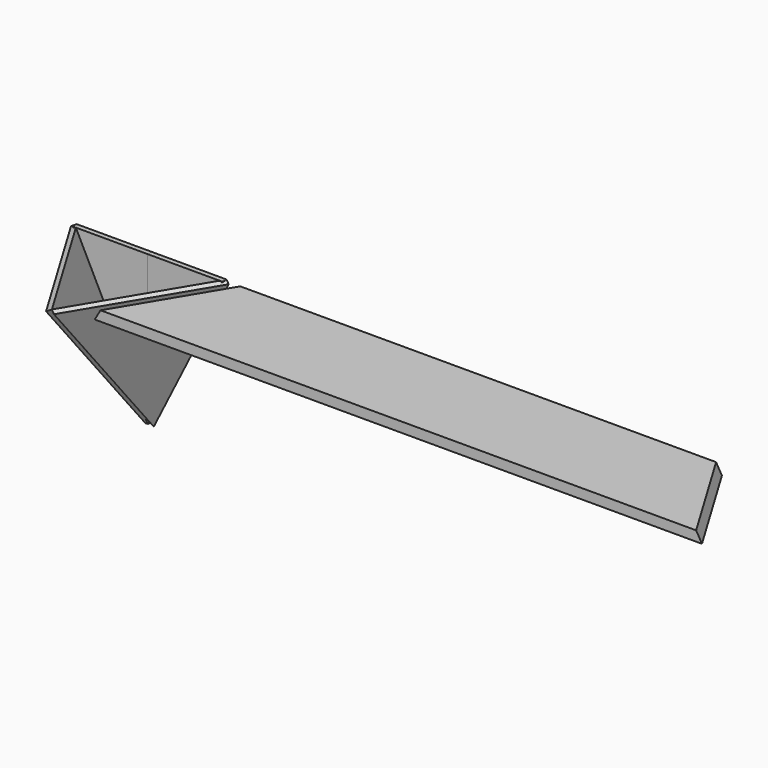
from build123d import *

# Parameters (mm, degrees)
F4_DEPTH     = 25.4
F5_DEPTH     = 25.4
F8_DEPTH     = 50.8
F9_T1_DEPTH  = 1118.6779391399
F10_T1_DEPTH = 1118.6779391399


# Not quite as in the source:
# - a fillet or chamfer that OpenCascade refuses, or shapes differently, is made with other operations: its cross-section is extruded or revolved along the edge and cut away or added


with BuildPart() as f4:
    # F3 (on 3pt) → F4 (new body)
    with BuildSketch(Plane(origin=(236.6459627329, -141.9875776398, -118.3229813665), x_dir=(0.4229444261, 0.8811342211, -0.2114722131), z_dir=(0.7881104062, -0.4728662437, -0.3940552031))):
        Polygon((161.141826348, -681.5535195419), (161.141826348, 170.3883798855), (-559.5202303749, 0), align=None)
    extrude(amount=F4_DEPTH)

    # F1 (on Front) → F5 (join)
    with BuildSketch(Plane.XZ):
        Polygon((381, 0), (0, 0), (0, -762), align=None)
    extrude(amount=F5_DEPTH)


with BuildPart() as f6_1:
    # F6: instance of F4
    add(f4.part.mirror(Plane.YZ))


with BuildPart() as f8:
    # F7 (on Top) → F8 (new body)
    with BuildSketch(Plane.XY):
        Polygon((2941.0180043185, -12.0108025911), (401.0180043185, -12.0108025911), (96.2180043185, -520.0108025911), (401.0180043185, -520.0108025911), (2941.0180043185, -520.0108025911), (3245.8180043185, -520.0108025911), align=None)
    extrude(amount=-F8_DEPTH)

    # F9: chamfer of 50.8 x 101.5999998984 on 1 edges, made by hand

    # F9_s2 → F9_t1 (cut)
    with BuildSketch(Plane(origin=(236.2304668654, 393.7174447757, 0), x_dir=(0, 0, 1), z_dir=(-0.5144957554, -0.8574929257, 0))):
        Polygon((0, -400.8496087388), (-101.5999998984, -350.0496087388), (0, -350.0496087388), align=None)
    extrude(amount=F9_T1_DEPTH, mode=Mode.SUBTRACT)

    # F10: chamfer of 50.8 x 101.5999998984 on 1 edges, made by hand

    # F10_s2 → F10_t1 (cut)
    with BuildSketch(Plane(origin=(1223.981175034, -2039.9686250567, 0), x_dir=(0, 0, 1), z_dir=(-0.5144957554, 0.8574929257, 0))):
        Polygon((0, 2464.9226261439), (-101.5999998984, 2515.7226261439), (0, 2515.7226261439), align=None)
    extrude(amount=F10_T1_DEPTH, mode=Mode.SUBTRACT)


solid = Compound([f4.part, f6_1.part, f8.part])
